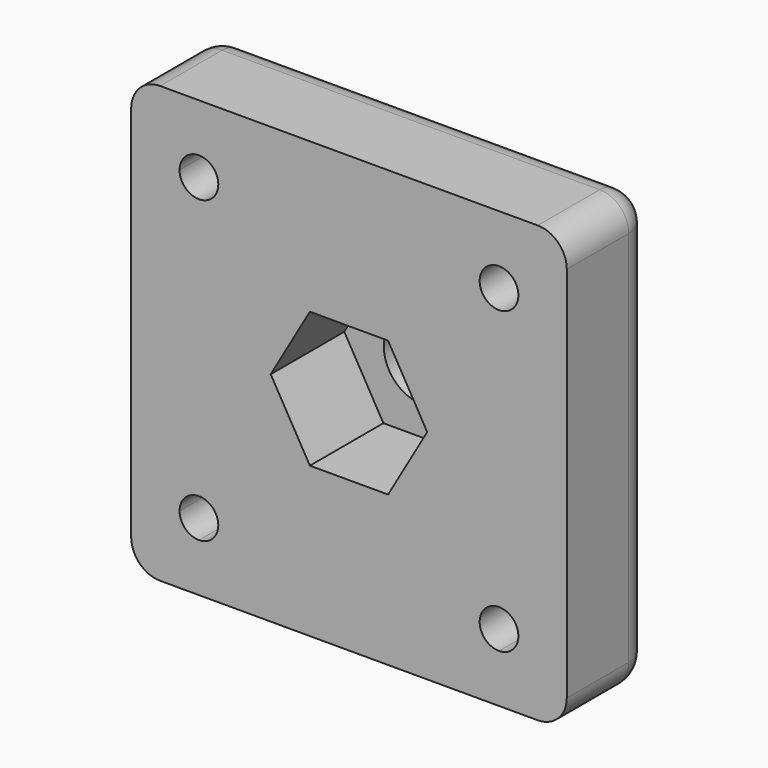
from build123d import *

# Parameters (mm, degrees)
F0_R     = 12.5
F0_R_2   = 4
F1_DEPTH = 11
F2_DEPTH = 15
F3_DEPTH = 9.5
F5_R     = 3
F6_SIZE  = 1.99999


# Not quite as in the source:
# - a fillet or chamfer that OpenCascade refuses, or shapes differently, is made with other operations: its cross-section is extruded or revolved along the edge and cut away or added
# - a fillet or chamfer is up to 0.001 mm smaller than in the source, because OpenCascade refuses the exact size


with BuildPart() as f1:
    # F0 (on Front) → F1 (new body)
    with BuildSketch(Plane.XZ):
        with BuildLine():
            Line((15.5, -22.5), (22.5, -22.5))
            Line((22.5, -22.5), (22.5, -15.5))
            Line((22.5, -15.5), (17.5, -15.5))
            ThreePointArc((17.5, -15.5), (16.9142135624, -16.9142135624), (15.5, -17.5))
            Line((15.5, -17.5), (15.5, -22.5))
        make_face()
        with BuildLine():
            Line((-15.5, -22.5), (15.5, -22.5))
            Line((15.5, -22.5), (15.5, -17.5))
            ThreePointArc((15.5, -17.5), (14.0857864376, -14.0857864376), (17.5, -15.5))
            Line((17.5, -15.5), (22.5, -15.5))
            Line((22.5, -15.5), (22.5, 15.5))
            Line((22.5, 15.5), (17.5, 15.5))
            ThreePointArc((17.5, 15.5), (14.0857864376, 14.0857864376), (15.5, 17.5))
            Line((15.5, 17.5), (15.5, 22.5))
            Line((15.5, 22.5), (-15.5, 22.5))
            Line((-15.5, 22.5), (-15.5, 17.5))
            ThreePointArc((-15.5, 17.5), (-14.0857864376, 16.9142135624), (-13.5, 15.5))
            ThreePointArc((-13.5, 15.5), (-15.5, 13.5), (-17.5, 15.5))
            Line((-17.5, 15.5), (-22.5, 15.5))
            Line((-22.5, 15.5), (-22.5, -15.5))
            Line((-22.5, -15.5), (-17.5, -15.5))
            ThreePointArc((-17.5, -15.5), (-15.5, -13.5), (-13.5, -15.5))
            ThreePointArc((-13.5, -15.5), (-14.0857864376, -16.9142135624), (-15.5, -17.5))
            Line((-15.5, -17.5), (-15.5, -22.5))
        make_face()
        Circle(F0_R, mode=Mode.SUBTRACT)
        with BuildLine():
            Line((-22.5, -22.5), (-15.5, -22.5))
            Line((-15.5, -22.5), (-15.5, -17.5))
            ThreePointArc((-15.5, -17.5), (-16.9142135624, -16.9142135624), (-17.5, -15.5))
            Line((-17.5, -15.5), (-22.5, -15.5))
            Line((-22.5, -15.5), (-22.5, -22.5))
        make_face()
        with BuildLine():
            Line((17.5, 15.5), (22.5, 15.5))
            Line((22.5, 15.5), (22.5, 22.5))
            Line((22.5, 22.5), (15.5, 22.5))
            Line((15.5, 22.5), (15.5, 17.5))
            ThreePointArc((15.5, 17.5), (16.9142135624, 16.9142135624), (17.5, 15.5))
        make_face()
        with BuildLine():
            Line((-22.5, 22.5), (-22.5, 15.5))
            Line((-22.5, 15.5), (-17.5, 15.5))
            ThreePointArc((-17.5, 15.5), (-16.9142135624, 16.9142135624), (-15.5, 17.5))
            Line((-15.5, 17.5), (-15.5, 22.5))
            Line((-15.5, 22.5), (-22.5, 22.5))
        make_face()
        Circle(F0_R)
        Polygon((8.0829037687, 0), (4.0414518843, -7), (-4.0414518843, -7), (-8.0829037687, 0), (-4.0414518843, 7), (4.0414518843, 7), align=None, mode=Mode.SUBTRACT)
        Polygon((-4.0414518843, -7), (4.0414518843, -7), (8.0829037687, 0), (4.0414518843, 7), (-4.0414518843, 7), (-8.0829037687, 0), align=None)
        Circle(F0_R_2, mode=Mode.SUBTRACT)
    extrude(amount=-F1_DEPTH)

    # F0 (on Front) → F2 (join)
    with BuildSketch(Plane.XZ):
        Circle(F0_R)
        Polygon((8.0829037687, 0), (4.0414518843, -7), (-4.0414518843, -7), (-8.0829037687, 0), (-4.0414518843, 7), (4.0414518843, 7), align=None, mode=Mode.SUBTRACT)
        Polygon((-4.0414518843, -7), (4.0414518843, -7), (8.0829037687, 0), (4.0414518843, 7), (-4.0414518843, 7), (-8.0829037687, 0), align=None)
        Circle(F0_R_2, mode=Mode.SUBTRACT)
    extrude(amount=-F2_DEPTH)

    # F0 (on Front) → F3 (cut)
    with BuildSketch(Plane.XZ):
        Polygon((-4.0414518843, -7), (4.0414518843, -7), (8.0829037687, 0), (4.0414518843, 7), (-4.0414518843, 7), (-8.0829037687, 0), align=None)
        Circle(F0_R_2, mode=Mode.SUBTRACT)
    extrude(amount=-F3_DEPTH, mode=Mode.SUBTRACT)

    # F4: fillet of radius 5 on 1 edges, made by hand

    # F4_s1 → F4_t2 (revolve)
    with BuildSketch(Plane.XY):
        with BuildLine():
            ThreePointArc((17.3989794856, 11), (14.2367018254, 12.1270166538), (12.5, 15))
            Line((12.5, 15), (12.5, 11))
            Line((12.5, 11), (17.3989794856, 11))
        make_face()
    revolve(axis=Axis((0, 11, 0), (0, -1, 0)))

    # F5
    f5_edges = [f1.edges().sort_by_distance(p)[0] for p in [
        (-12.5, 15, 0),
        (0, 11, -22.5),
        (-22.5, 11, 0),
        (-22.5, 5.5, -22.5),
        (-22.5, 5.5, 22.5),
        (0, 11, 22.5),
        (22.5, 5.5, 22.5),
        (22.5, 11, 0),
        (22.5, 5.5, -22.5),
    ]]
    fillet(f5_edges, radius=F5_R)

    # F6 (size 2 in the source; OpenCascade refuses exactly that, so slightly less here)
    f6_edges = [f1.edges().sort_by_distance(p)[0] for p in [
        (-13.5, 11, 15.5),
        (-15.5, 11, -13.5),
        (15.5, 11, -13.5),
        (15.5, 11, 13.5),
    ]]
    chamfer(f6_edges, length=F6_SIZE)


solid = f1.part
